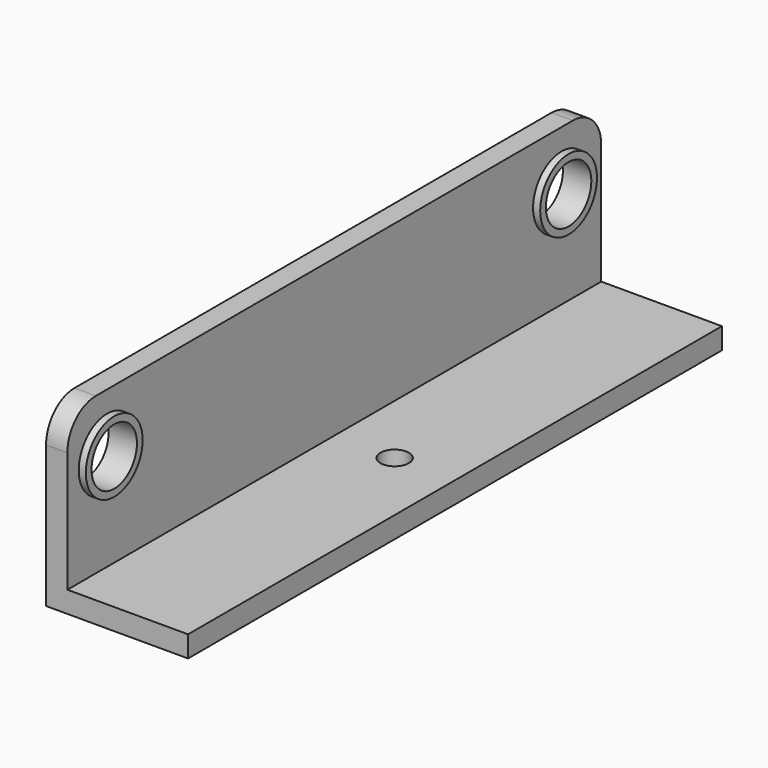
from build123d import *

# Parameters (mm, degrees)
F0_W     = 20
F0_H     = 94
F1_DEPTH = 25
F2_R     = 5
F2_R_2   = 4
F3_DEPTH = 17
F4_DEPTH = 20
F5_START = -16
F5_DEPTH = 1
F6_R     = 5
F7_R     = 2
F8_DEPTH = 3


# Not quite as in the source:
# - a pattern or mirror of a feature is missing from the dataset's text; its kind, count and spacing are read off the source's solid


with BuildPart() as f1:
    # F0 (on Top) → F1 (new body)
    with BuildSketch(Plane.XY):
        with Locations((-55, 0)):
            Rectangle(F0_W, F0_H)
    extrude(amount=F1_DEPTH)

    # F2 (on face) → F3 (cut)
    with BuildSketch(Plane.YZ.offset(-45)):
        with BuildLine():
            Line((-32.4501655647, 25), (-47, 25))
            Line((-47, 25), (-47, 8.5147186258))
            ThreePointArc((-47, 8.5147186258), (-35.3095842402, 7.0501256289), (-29, 17))
            ThreePointArc((-29, 17), (-29.8993025293, 21.3561348241), (-32.4501655647, 25))
        make_face()
        with Locations((-40, 17)):
            Circle(F2_R, mode=Mode.SUBTRACT)
        with BuildLine():
            Line((-29.753049234, 25), (-32.4501655647, 25))
            ThreePointArc((-32.4501655647, 25), (-29.8993025293, 21.3561348241), (-29, 17))
            ThreePointArc((-29, 17), (-35.3095842402, 7.0501256289), (-47, 8.5147186258))
            Line((-47, 8.5147186258), (-47, 6.0455488499))
            ThreePointArc((-47, 6.0455488499), (-33.7550020016, 5.598245749), (-27, 17))
            ThreePointArc((-27, 17), (-27.7075153049, 21.2302269468), (-29.753049234, 25))
        make_face()
        with BuildLine():
            Line((47, 25), (-29.753049234, 25))
            ThreePointArc((-29.753049234, 25), (-27.7075153049, 21.2302269468), (-27, 17))
            ThreePointArc((-27, 17), (-33.7550020016, 5.598245749), (-47, 6.0455488499))
            Line((-47, 6.0455488499), (-47, 3))
            Line((-47, 3), (47, 3))
            Line((47, 3), (47, 25))
        make_face()
        with Locations((-40, 17)):
            Circle(F2_R)
        with Locations((-40, 17)):
            Circle(F2_R_2, mode=Mode.SUBTRACT)
    extrude(amount=-F3_DEPTH, mode=Mode.SUBTRACT)

    # F2 (on face) → F4 (cut, through all)
    with BuildSketch(Plane.YZ.offset(-45)):
        with Locations((-40, 17)):
            Circle(F2_R_2)
    f4 = extrude(amount=-F4_DEPTH, mode=Mode.SUBTRACT)

    # F4_copies: F4 across plane
    add(f4.mirror(Plane.ZX), mode=Mode.SUBTRACT)

    # F2 (on face) → F5 (join)
    with BuildSketch(Plane.YZ.offset(-45).offset(F5_START)):
        with Locations((-40, 17)):
            Circle(F2_R)
        with Locations((-40, 17)):
            Circle(F2_R_2, mode=Mode.SUBTRACT)
    f5 = extrude(amount=-F5_DEPTH)

    # F5_copies: F5 across plane
    add(f5.mirror(Plane.ZX))

    # F6
    f6_edges = [f1.edges().sort_by_distance(p)[0] for p in [
        (-63.5, -47, 25),
        (-63.5, 47, 25),
    ]]
    fillet(f6_edges, radius=F6_R)

    # F7 (on face) → F8 (cut, through all)
    with BuildSketch(Plane.XY.offset(3)):
        with Locations((-53.5, 0)):
            Circle(F7_R)
    extrude(amount=-F8_DEPTH, mode=Mode.SUBTRACT)


solid = f1.part
